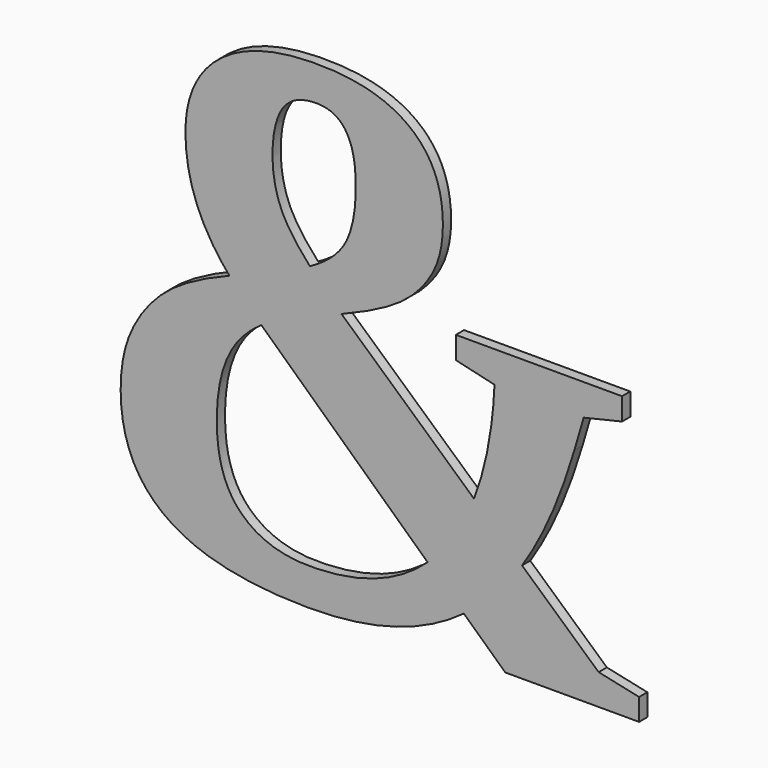
from build123d import *

# Parameters (mm, degrees)
F0_TEXT_SIZE = 694.4444444444
F1_DEPTH     = 10


# Not quite as in the source:
# - Text() gives the source's letters only with a copy of the font that has no kerning and outlines rounded to 1/6400 em; it was checked with that copy


with BuildPart() as f1:
    # F0 (on Front) → F1 (new body)
    with BuildSketch(Plane.XZ):
        with Locations((-372.7544663328, -261.9760457925)):
            Text('&', F0_TEXT_SIZE, font='Tinos', font_style=FontStyle.BOLD, text_align=(TextAlign.LEFT, TextAlign.BOTTOM))
    extrude(amount=F1_DEPTH)


solid = f1.part
